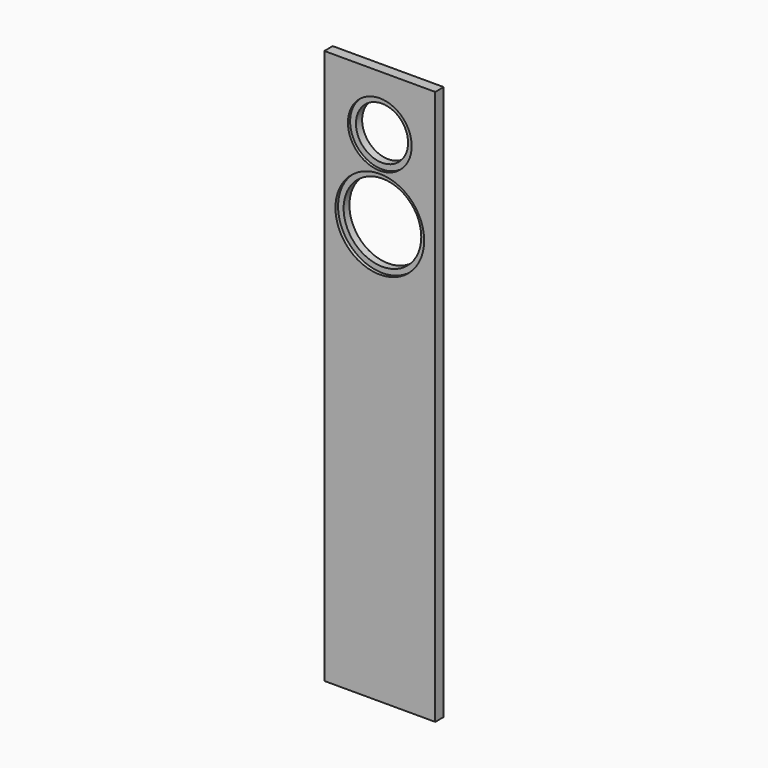
from build123d import *

# Parameters (mm, degrees)
F0_W     = 200
F0_H     = 1000
F1_DEPTH = 19
F2_R     = 57.5
F3_DEPTH = 5
F4_R     = 47
F5_DEPTH = 25
F6_R     = 80
F7_DEPTH = 6
F8_R     = 70
F9_DEPTH = 25


# Not quite as in the source:
# - a feature names something its author has since deleted; it is built from what else it names


with BuildPart() as f1:
    # F0 (on Front) → F1 (new body)
    with BuildSketch(Plane.XZ):
        Rectangle(F0_W, F0_H)
    extrude(amount=F1_DEPTH)

    # F2 (on face) → F3 (cut)
    with BuildSketch(Plane.XZ.offset(19)):
        with Locations((0, 400)):
            Circle(F2_R)
    extrude(amount=-F3_DEPTH, mode=Mode.SUBTRACT)

    # F4 (on face) → F5 (cut)
    with BuildSketch(Plane.XZ.offset(19)):
        with Locations((0, 400)):
            Circle(F4_R)
    extrude(amount=-F5_DEPTH, mode=Mode.SUBTRACT)

    # F6 (on face) → F7 (cut)
    with BuildSketch(Plane.XZ.offset(19)):
        with Locations((0, 257.5)):
            Circle(F6_R)
    extrude(amount=-F7_DEPTH, mode=Mode.SUBTRACT)

    # F8 (on face) + F0 (on Front) → F9 (cut)
    with BuildSketch(Plane.XZ.offset(19)):
        with Locations((0, 257.5)):
            Circle(F8_R)
    with BuildSketch(Plane.XZ):
        Rectangle(F0_W, F0_H)
    extrude(amount=-F9_DEPTH, mode=Mode.SUBTRACT)


solid = f1.part
